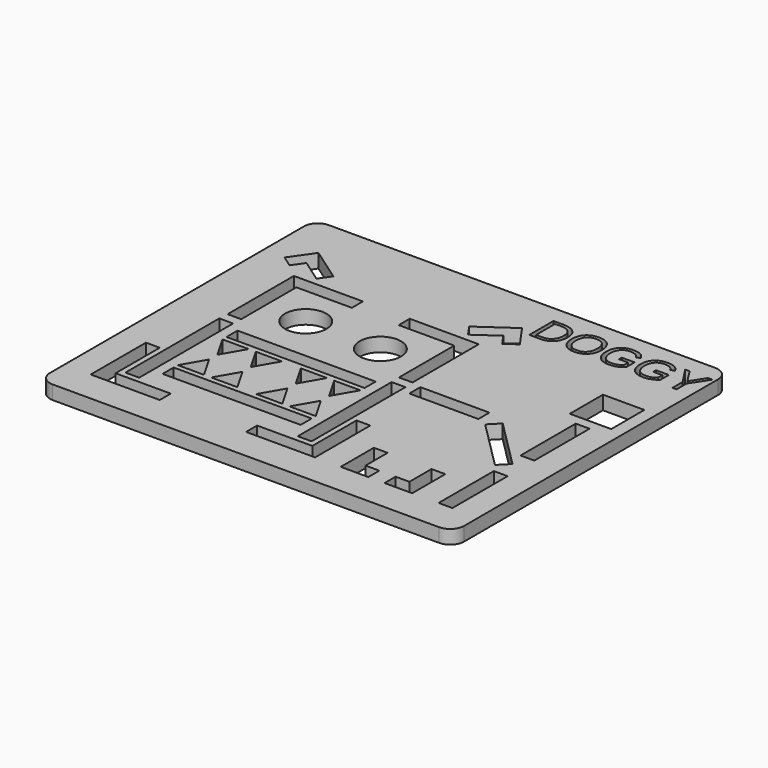
from build123d import *

# Parameters (mm, degrees)
F1_DEPTH     = 10
F2_W         = 50
F2_H         = 10
F2_W_2       = 10
F2_H_2       = 50
F2_H_3       = 85
F2_R         = 15
F2_W_3       = 30
F2_H_4       = 30
F2_TEXT_SIZE = 31.8302387268
F3_DEPTH     = 10


# Not quite as in the source:
# - Text() gives the source's letters only with a copy of the font that has no kerning and outlines rounded to 1/6400 em; it was checked with that copy


with BuildPart() as f1:
    # F0 (on Top) → F1 (new body)
    with BuildSketch(Plane.XY):
        with BuildLine():
            Line((140, 125), (-140, 125))
            ThreePointArc((-140, 125), (-147.0710678119, 122.0710678119), (-150, 115))
            Line((-150, 115), (-150, -115))
            ThreePointArc((-150, -115), (-147.0710678119, -122.0710678119), (-140, -125))
            Line((-140, -125), (140, -125))
            ThreePointArc((140, -125), (147.0710678119, -122.0710678119), (150, -115))
            Line((150, -115), (150, 115))
            ThreePointArc((150, 115), (147.0710678119, 122.0710678119), (140, 125))
        make_face()
    extrude(amount=F1_DEPTH)

    # F2 (on face) → F3 (cut)
    with BuildSketch(Plane.XY.offset(10)):
        with Locations((49.4691804051, -2.6507945731)):
            Rectangle(F2_W, F2_H)
        with Locations((126.1362165958, -76.9677194953)):
            Rectangle(F2_W_2, F2_H_2)
        Polygon((123.992735641, -38.6448626873), (88.6373965817, -3.2895236279), (81.5663287698, -10.3605914398), (116.9216678292, -45.7159304991), align=None)
        with Locations((-111.9676977396, -45.4465248622)):
            Rectangle(F2_W_2, F2_H_3)
        Polygon((-116.5110979927, 4.016289141), (-106.6892413194, 4.016289141), (-106.6892413194, 54.016289141), (-66.5110979927, 54.0162891412), (-66.5110979927, 64.0162891412), (-116.5110979927, 64.0162891412), align=None)
        Polygon((-120.8139190078, -52.0559701137), (-130.8139190078, -52.0559701137), (-130.8139190078, -102.0559701137), (-120.8139190078, -102.0559701137), (-80.8139190078, -102.0559701137), (-80.8139190078, -92.0559701137), (-120.8139190078, -92.0559701137), align=None)
        Polygon((-32.5770418393, 54.0162891412), (7.6011014873, 54.016289141), (7.6011014873, 4.016289141), (17.4229581607, 4.016289141), (17.4229581607, 64.0162891412), (-32.5770418393, 64.0162891412), align=None)
        with Locations((12.8795579076, -45.4465248622)):
            Rectangle(F2_W_2, F2_H_3)
        Polygon((21.7257791758, -52.0559701137), (21.7257791758, -92.0559701137), (-18.2742208242, -92.0559701137), (-18.2742208242, -102.0559701137), (31.7257791758, -102.0559701137), (31.7257791758, -52.0559701137), align=None)
        with Locations((-74.544069916, -13.1720205583)):
            Rectangle(F2_W, F2_H)
        with Locations((-24.544069916, -71.0433196463)):
            Rectangle(F2_W, F2_H)
        with Locations((-74.544069916, -71.0433196463)):
            Rectangle(F2_W, F2_H)
        with Locations((-24.544069916, -13.1720205583)):
            Rectangle(F2_W, F2_H)
        with Locations((-76.5782669187, 24.8359744437)):
            Circle(F2_R)
        with Locations((-22.5098729134, 24.8359744437)):
            Circle(F2_R)
        Polygon((70.279174, -102.0534406416), (70.279174, -92.0534406416), (60.279174, -92.0534406416), (60.279174, -72.0534406416), (50.279174, -72.0534406416), (50.279174, -102.0534406416), align=None)
        Polygon((82.0438414812, -92.0534369163), (82.0438414812, -102.0534369163), (102.0438414812, -102.0534369163), (102.0438414812, -72.0534369163), (92.0438414812, -72.0534369163), (92.0438414812, -92.0534369163), align=None)
        Polygon((-134.7594320955, 78.3937743621), (-126.5679116526, 72.6580099986), (-120.8321472891, 80.8495304415), (-104.4491064033, 69.3780017144), (-98.7133420398, 77.5695221573), (-123.2879033685, 94.7768152479), align=None)
        Polygon((-99.5002330731, -21.8885384966), (-90.0005847216, -38.3424120955), (-80.50093637, -21.8885384966), align=None)
        Polygon((-75.3332914304, -21.8885384966), (-65.8336430788, -38.3424120955), (-56.3339947272, -21.8885384966), align=None)
        Polygon((-33.2544967532, -38.3424120955), (-23.7548484017, -21.8885384966), (-42.7541451048, -21.8885384966), align=None)
        Polygon((-18.587203462, -21.8885384966), (-9.0875551105, -38.3424120955), (0.4120932411, -21.8885384966), align=None)
        Polygon((-80.50093637, -62.326801708), (-90.0005847216, -45.872928109), (-99.5002330731, -62.326801708), align=None)
        Polygon((-56.3339947272, -62.326801708), (-65.8336430788, -45.872928109), (-75.3332914304, -62.326801708), align=None)
        Polygon((-42.7541451048, -62.326801708), (-23.7548484017, -62.326801708), (-33.2544967532, -45.872928109), align=None)
        Polygon((0.4120932411, -62.326801708), (-9.0875551105, -45.872928109), (-18.587203462, -62.326801708), align=None)
        Polygon((35.6712922635, 78.3937743621), (24.1997635365, 94.7768152479), (-0.3747977922, 77.5695221573), (5.3609665713, 69.3780017144), (21.7440074571, 80.8495304415), (27.4797718206, 72.6580099986), align=None)
        with Locations((126.005589962, -2.6535177603)):
            Rectangle(F2_W_2, F2_H_2)
        with Locations((125.8478978276, 44.6810232103)):
            Rectangle(F2_W_3, F2_H_4)
        with Locations((30, 90.8145938395)):
            Text('DOGGY', F2_TEXT_SIZE, font='Arimo', text_align=(TextAlign.LEFT, TextAlign.BOTTOM))
    extrude(amount=-F3_DEPTH, mode=Mode.SUBTRACT)


solid = f1.part
